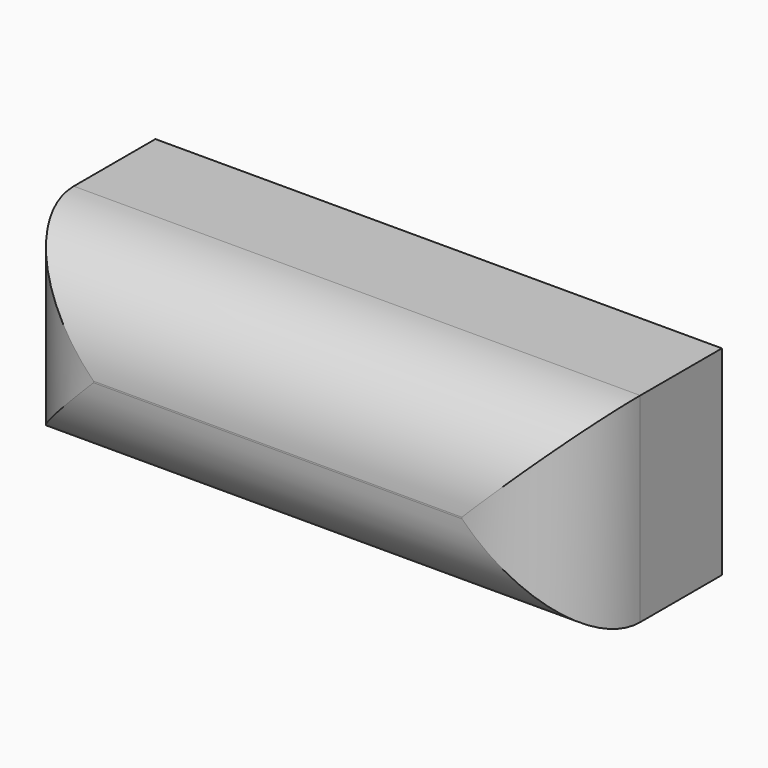
from build123d import *

# Parameters (mm, degrees)
F0_W     = 47.9163888
F0_H     = 16.881729
F1_DEPTH = 12.7
F2_R     = 8.382
F3_SIZE  = 8.382


# Not quite as in the source:
# - a feature names something its author has since deleted; it is built from what else it names


with BuildPart() as f1:
    # F0 (on Front) → F1 (new body, symmetric)
    with BuildSketch(Plane.XZ):
        Rectangle(F0_W, F0_H)
    extrude(amount=F1_DEPTH, both=True)

    # F2
    f2_edges = [f1.edges().sort_by_distance(p)[0] for p in [
        (0, -12.7, 8.440864),
        (0, -12.7, -8.440865),
        (-23.958194, -12.7, 0),
        (23.958194, -12.7, 0),
    ]]
    fillet(f2_edges, radius=F2_R)

    # F3
    f3_edges = [f1.edges().sort_by_distance(p)[0] for p in [
        (0, 12.7, 8.440864),
        (23.958194, 12.7, 0),
        (0, 12.7, -8.440865),
        (-23.958194, 12.7, 0),
    ]]
    chamfer(f3_edges, length=F3_SIZE)


solid = f1.part
